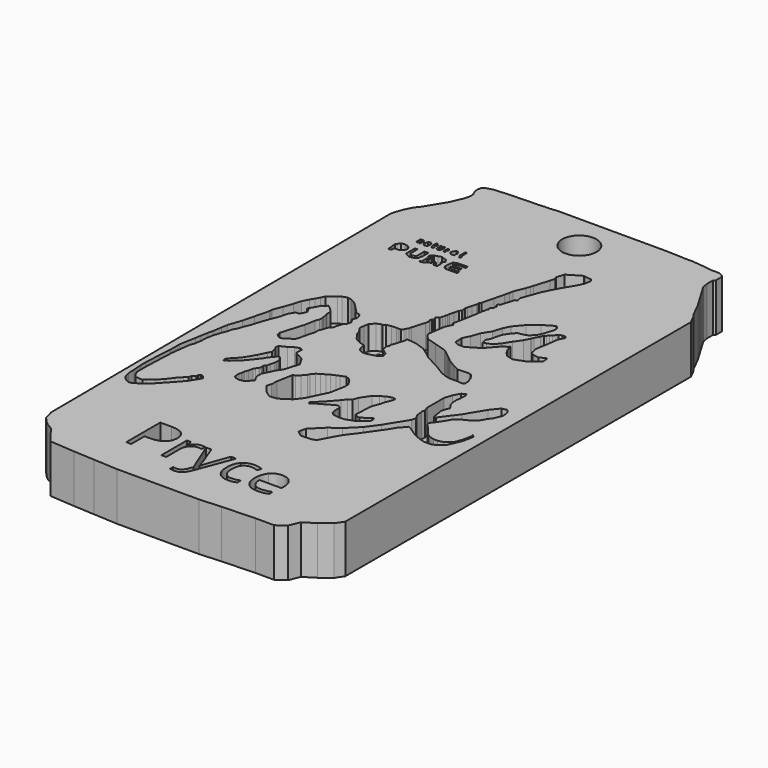
from build123d import *

# Parameters (mm, degrees)
F0_TEXT_SIZE = 6.2945538149
F1_DEPTH     = 2.54
F0_R         = 1.81247456
F2_DEPTH     = 5.08


# Not quite as in the source:
# - Text() gives the source's letters only with a copy of the font that has no kerning and outlines rounded to 1/6400 em; it was checked with that copy


with BuildPart() as f1:
    # F0 (on Top) → F1 (new body)
    with BuildSketch(Plane.XY):
        with Locations((-18.4478778392, -11.3192549907)):
            Text('Pryce', F0_TEXT_SIZE, font='Open Sans', text_align=(TextAlign.LEFT, TextAlign.BOTTOM))
        Polygon((-14.624286443, 6.6065290011), (-14.6113066003, 6.5750698559), (-14.9114299302, 4.9573605225), (-14.9448718876, 4.2598485015), (-15.1049830019, 3.7795153912), (-14.4143942744, 2.9255894478), (-13.7573806569, 2.4585989304), (-13.0635658279, 2.5119693018), (-12.5832324848, 2.7521359734), (-11.8360472843, 3.2724970952), (-11.2489731982, 4.0330248885), (-10.6618991122, 5.2605429664), (-10.2616213262, 6.0610985383), (-10.065051727, 7.1206378795), (-9.9613657221, 7.6809348539), (-9.9613657221, 8.0247446895), (-9.9935978651, 8.2181375474), (-10.3374077007, 8.7553402409), (-10.6274969876, 9.0131983161), (-10.9498184174, 9.142126888), (-11.4547898993, 8.9487340301), (-11.7878550664, 8.7983170524), (-12.1961291879, 8.626411669), (-12.5399390236, 8.4115304053), (-12.9267256707, 8.2181375474), (-13.2705355063, 7.9817688093), (-13.5713685304, 7.6164705679), (-13.6788096279, 7.42307771), (-14.0441069379, 6.9825709797), (-14.3879167736, 6.6924816929), align=None)
        Polygon((-13.0409123376, 6.1027472839), (-13.0857918411, 6.4729987644), (-13.0801750347, 6.4761852846), (-13.0689619109, 6.433729548), (-12.9118859768, 6.568366196), (-12.9343252629, 6.7030033097), (-12.9343252629, 6.7927609198), (-12.6426117495, 7.0171556436), (-12.205041945, 6.9947163574), (-11.9582079351, 6.9498373196), (-11.7450328544, 6.8376399577), (-11.5206381306, 6.568366196), (-11.3635621965, 6.489828229), (-11.3523425534, 6.2934826128), (-11.3579519093, 5.9400605969), (-11.3803921267, 5.8390833437), (-11.4028314129, 5.682006944), (-11.4925885573, 5.4744416848), (-11.5150287747, 5.4127331823), (-11.6496654227, 5.1434594207), (-12.0984548703, 4.6722302213), (-12.2555308044, 4.4702752493), (-12.3004103079, 4.3917368166), (-12.3901683837, 4.2234407738), (-12.5696836039, 3.9766067639), (-12.6987108961, 3.920508083), (-12.9511551932, 3.987826407), (-13.197989203, 4.2234412394), (-13.3101865649, 4.3973471038), (-13.2821369916, 4.6329614706), (-13.2540874183, 4.9639437348), (-13.0970114842, 5.2163880318), (-13.18676956, 5.2163880318), (-13.197989203, 5.3229755722), (-13.0745721981, 5.4407827556), align=None, mode=Mode.SUBTRACT)
        Polygon((-20.1555043459, 6.0734697618), (-20.7176841795, 5.5137774907), (-20.754635334, 5.265337415), (-20.6640698016, 5.0563374534), (-20.3923713416, 5.265337415), (-20.2739369124, 5.3280373104), (-20.0928039849, 5.5161374621), (-19.6121055633, 5.9132371098), (-19.4518715143, 6.0804365203), (-19.2777048796, 6.2964032404), (-18.9781393856, 6.6517028026), (-18.671605736, 7.0279026404), (-18.5253061354, 7.2438688949), (-18.3650720865, 7.4389353395), (-18.3650720865, 7.4946684763), (-18.0794391781, 7.8778350726), (-17.5848063082, 8.4909005091), (-17.4036733806, 8.4212338552), (-17.1110741794, 8.0032348633), (-17.1110741794, 7.8360345215), (-17.1110741794, 7.6131019741), (-17.1389412135, 7.3901684955), (-17.2583172873, 7.020606572), (-17.3409748822, 6.5750698559), (-17.5290741026, 6.3939369284), (-17.5012070686, 6.1222370714), (-17.5639074296, 5.8784037828), (-17.75200665, 5.6276042014), (-17.8704392165, 5.4325377569), (-17.9540403187, 4.9588046968), (-18.0028062314, 4.8473384231), (-18.0794391781, 4.6244054101), (-18.114272505, 4.457205534), (-18.1351732463, 4.2551723309), (-18.1909073144, 4.0252725594), (-18.2187724859, 3.7326728925), (-18.1769728661, 3.6421061959), (-18.1630402803, 3.4540065099), (-17.9819073528, 3.3007399179), (-17.7589729428, 3.2241067383), (-17.4454730004, 3.1962399371), (-17.1423219144, 3.2592936148), (-16.3936476487, 3.8831883856), (-16.4492409676, 3.9765057154), (-16.6443083435, 4.2760721408), (-16.7766753584, 4.6522719786), (-16.7740557998, 5.187679922), (-16.4422746748, 5.8366036974), (-16.2193421274, 6.3591031358), (-15.8156915272, 6.9102430428), (-15.5505435541, 7.7872681431), (-15.3276110068, 8.4560671821), (-15.8292111009, 9.3129668385), (-16.1636099219, 9.5358993858), (-16.5398102254, 9.7100660205), (-16.8602764606, 9.9120996892), (-16.8254431337, 10.6366323307), (-17.083209008, 10.7480986044), (-17.5778418779, 10.6017990038), (-18.0585421622, 10.2743655443), (-18.7552068383, 9.9329994991), (-18.8109409064, 9.5985997468), (-18.6642110338, 9.453726537), (-18.5322742909, 8.7695671245), (-18.7203735113, 8.4421345964), (-19.1244389862, 7.5991684571), (-19.7096392512, 6.6308025271), align=None)
        Polygon((-20.4632785171, 17.7643876523), (-20.2095806599, 17.9161417095), (-20.0275518, 18.1322433054), (-19.7358392179, 17.9161417095), (-19.3880274892, 17.5712574273), (-19.2085113376, 17.3917412758), (-19.2197300494, 16.9373415411), (-19.1243626177, 16.6400186718), (-19.0963130444, 16.3146462291), (-19.0417472463, 16.0316946908), (-19.0738718957, 15.7312210649), (-19.2253384739, 15.3273111209), (-19.4257468986, 14.2470799403), (-20.1641112822, 11.804805575), (-20.1018537056, 11.4819682355), (-19.9315026402, 11.3378688693), (-19.6667686105, 11.1288689077), (-19.3184353411, 11.2124690786), (-19.0397705883, 11.3587686792), (-18.8656039536, 11.5468688309), (-18.6496376991, 11.6165354848), (-18.3849036694, 11.895201169), (-18.196804449, 12.7312000841), (-18.0087033659, 13.4487664327), (-17.9181378335, 13.6508001015), (-17.9383958732, 14.1109345587), (-17.7718382329, 14.5355658606), (-17.5837371498, 15.0928990915), (-17.3062126196, 15.3241693663), (-17.231864767, 15.7249153367), (-17.0542709529, 16.2702649832), (-16.8104376644, 16.5419634432), (-16.7129039764, 16.9878304005), (-16.9183981761, 17.3327669933), (-17.0055031776, 17.3709969968), (-16.7895369232, 17.9161417095), (-16.9776361436, 18.4020623565), (-17.1796698123, 18.5553282499), (-17.4722690135, 18.5135286301), (-17.5976697356, 18.7573619187), (-18.653165549, 19.8301617056), (-19.2760806531, 20.1762262732), (-19.6913573891, 20.2454384416), (-20.2018022537, 20.0897101313), (-20.5046068877, 19.8993738741), (-21.2585731294, 19.2710691265), (-21.4562844485, 18.8265759498), (-21.6985289007, 18.4112992138), (-21.9321213663, 18.0219765753), (-22.2736951587, 17.3538995261), (-22.4944781512, 16.5771618485), (-22.8405427188, 15.6341381371), (-23.2212133706, 14.6392034367), (-23.2212133706, 14.3277458847), (-23.6091244797, 12.8109433288), (-23.914789253, 11.6157388134), (-24.3805292994, 10.2355387062), (-24.5034418927, 9.5730215691), (-24.6367733926, 8.6511746049), (-24.7707884197, 8.1271516241), (-24.9091346494, 7.3814448938), (-24.9975714833, 6.7610526457), (-25.3097963567, 5.0781141951), (-25.3097963567, 3.8123764098), (-25.4116076976, 2.5146363769), (-25.4894718528, 0.8456546348), (-25.4894718528, 0.1838220051), (-25.4116076976, -0.8108470356), (-25.3763237316, -1.6122754474), (-25.2426378429, -2.1516056731), (-24.9677542597, -2.5162470993), (-24.4183161264, -2.845908402), (-24.0084677935, -2.7518614661), (-23.6438252032, -2.5050272234), (-23.2904031873, -2.2357534617), (-22.6845387369, -1.7813541926), (-21.1651660502, -0.1317714487), (-20.6806752831, 0.4392341943), (-20.1382439994, 1.3322597274), (-20.0145021081, 1.5466390178), (-20.1875343919, 1.7975354567), (-20.3346125782, 1.8927031197), (-20.5422509462, 1.9100062782), (-20.6806752831, 1.7629291397), (-20.6806752831, 1.5293358592), (-20.7498893142, 1.4255166752), (-21.0094377398, 1.2438331032), (-21.0786499083, 0.9323754348), (-21.3728044182, 0.6987822126), (-21.8572933227, 0.1796862052), (-22.376390174, -0.5124418531), (-22.9560472071, -1.118053915), (-23.5097501427, -1.585240243), (-23.7450870523, -1.7813541926), (-24.5411440238, -1.7189012933), (-24.7647128999, -1.4563115546), (-24.9795932323, -0.9728290606), (-24.9795932323, -0.4893464502), (-24.9795932323, 0.316457852), (-24.8936414719, 2.5146363769), (-24.8506646603, 3.4429784864), (-24.6014371514, 5.4905763827), (-24.429531768, 5.9310826473), (-24.300603196, 6.7261429504), (-24.300603196, 7.2203697637), (-24.1470049222, 8.0482872776), (-23.8063763827, 9.1005796567), (-23.6749453002, 9.3576429668), (-23.623727262, 9.6055511385), (-23.5914960504, 9.841920808), (-23.3658701181, 10.1964743808), (-23.1187567115, 10.8948387206), (-22.9038763791, 11.3890646026), (-22.6204795463, 12.3101534486), (-22.3344415426, 13.1296021864), (-21.9321213663, 14.1395442188), (-21.7650067061, 14.8701397702), (-21.4038180918, 15.4721236742), (-20.9914352745, 15.5147835612), (-20.6906013191, 16.1594264209), (-20.948458463, 16.6751425713), (-21.0988745093, 16.6536532342), (-20.6866535317, 17.340691484), align=None)
        Polygon((-9.5739997969, 4.6030381121), (-10.4910627902, 3.6900329869), (-10.4620512575, 3.5761527251), (-10.4620512575, 3.5200540442), (-10.3666838259, 3.5312739201), (-10.2769257501, 3.5761527251), (-10.1254591718, 3.688350087), (-9.8730148748, 3.8454264868), (-9.6934996545, 3.95201426), (-9.3681272119, 4.1259201244), (-8.7678711861, 4.4737318531), (-8.6220148951, 4.5522698201), (-8.3863995969, 4.664467182), (-8.2517629489, 4.6869069338), (-8.0161485821, 4.5747095719), (-7.9488297924, 4.4288528152), (-7.9376101494, 4.1820188053), (-7.9488297924, 3.9912830107), (-7.8927315772, 3.677130444), (-7.859072648, 3.4527357202), (-7.6056825928, 3.2059017103), (-7.5108190067, 3.1607286073), (-7.307539694, 3.129107412), (-7.0455353707, 3.0974859837), (-6.7564267665, 3.079416696), (-6.2685562298, 3.129107412), (-5.9162052348, 3.2781788614), (-5.4804068059, 3.4207922872), (-5.2138781175, 3.6071261857), (-4.7017219476, 4.004185088), (-4.4716764241, 4.2033214122), (-4.4438098557, 4.4819880277), (-4.5204432681, 4.7745876946), (-4.7224764712, 4.7188540921), (-4.9941758625, 4.4401879422), (-5.1962090656, 4.356588237), (-5.5793751962, 4.119721707), (-5.8092749678, 4.1475882754), (-6.1436747201, 4.356588237), (-6.0740080662, 6.1191529967), (-5.9486082755, 6.5650194883), (-5.7256752625, 7.1502188221), (-5.6420755573, 7.4985516258), (-5.5236420594, 7.8190183267), (-5.4191425443, 8.0349845812), (-5.3285756148, 8.3763506263), (-5.3285756148, 8.5435509682), (-5.5306088179, 8.6271502078), (-5.8859083802, 8.5644507781), (-6.2830080278, 8.3763506263), (-6.673140917, 8.1673506647), (-7.1735936217, 7.7911512926), (-7.8087067232, 6.8297521211), (-8.0177066848, 6.3072526827), (-8.3590727299, 6.0216202401), (-8.6934724823, 5.6036203168), align=None)
        Polygon((-6.4959203971, 1.0680862335), (-7.7450601384, -0.1755262492), (-7.8824013472, -0.5878285156), (-7.8914361075, -0.9853526717), (-7.575223688, -1.2563917553), (-7.2770807892, -1.428049989), (-6.6536907107, -1.3964286773), (-6.0845082626, -1.3467381941), (-5.7482607663, -1.1509091128), (-5.6089274585, -0.8583095041), (-5.2675609477, -0.2173767425), (-4.8843948171, 0.479289185), (-4.4716764241, 1.1202218011), (-3.9090625942, 1.8447544426), (-2.4584615603, 3.9023284335), (-1.9673923962, 4.6953144483), (-1.5308865113, 5.1827458665), (-1.3781094458, 5.382811185), (-1.1453062762, 5.3136977367), (-0.5341977812, 4.8808292486), (0.0550852492, 4.5097991824), (0.808058132, 4.2006075382), (1.0808744701, 4.1387691163), (1.2409265619, 4.069655668), (1.4519045362, 4.069655668), (1.6919827322, 4.069655668), (2.0157247782, 4.0805684403), (2.3649295326, 4.2033214122), (2.5940951891, 4.3788473122), (3.0742518138, 4.7426023521), (3.387081204, 5.4191863164), (3.7071856204, 6.1576091684), (3.8672378287, 6.9069443271), (3.9108884521, 7.1797608398), (3.9145257324, 7.3361755349), (3.6562599707, 7.5544281863), (3.7362859584, 7.3085627519), (3.5494896583, 6.3745812513), (3.2559528481, 5.574026145), (2.9357306194, 5.3071742877), (2.5621380191, 5.0403224304), (2.0284343045, 4.9202390946), (1.6014714492, 4.9335816875), (1.1211381061, 5.080350209), (0.6941751344, 5.3472020663), (0.004460323, 6.2304427847), (-0.2592035162, 6.4828866161), (-0.4331094678, 6.7072813399), (-0.5092399145, 6.951796861), (-0.3096923756, 7.1504614316), (0.3747116425, 8.1602381542), (0.6495952257, 8.653906174), (1.1097851675, 9.0257488191), (2.0230300725, 9.4877434894), (2.4742805399, 9.8852738738), (2.8288345784, 10.4869408533), (3.1619002111, 10.9596792608), (3.5057100467, 11.8192043155), (3.3767814748, 12.5068239868), (3.0974359252, 12.8076579422), (2.5709769689, 12.7002168447), (1.8511251546, 11.8084605783), (0.6692788447, 9.8422979936), (-0.6457643467, 8.0773709342), (-0.8101447602, 8.0341128632), (-0.8534026565, 8.1119779497), (-0.88800909, 8.1811901182), (-1.0437379824, 9.2539889738), (-0.9053121903, 9.8336460069), (-0.7322800811, 10.0499354303), (-1.130253775, 10.620941408), (-1.2340729591, 10.9670050442), (-1.2686793925, 11.6331782192), (-1.1994665256, 11.9532877579), (-1.156208571, 12.6454159617), (-1.3032857096, 12.9136154428), (-1.683956245, 12.680022046), (-2.047323389, 12.0225008577), (-2.306871349, 11.2179024145), (-2.306871349, 10.5776842684), (-2.306871349, 9.3837631866), (-2.306871349, 9.0030925348), (-2.151142573, 8.5359057412), (-2.211703686, 8.1552360207), (-2.1259179339, 7.4634985067), (-1.8573165871, 6.969272159), (-1.9540130161, 6.4965337515), (-3.3292525914, 4.2725135572), (-4.2559751181, 3.0073651436), (-5.4673198611, 1.801380422), align=None)
        Polygon((-8.3126790669, 34.6074029803), (-8.5634384304, 33.7779708207), (-8.4576277141, 33.6387456779), (-8.4563963125, 33.4593554644), (-8.565570089, 33.0324662643), (-9.0527144692, 31.4491625604), (-9.1438563541, 31.1476942152), (-9.2830456478, 30.7437833399), (-9.7441114485, 29.5993704349), (-9.8226498812, 29.2235091329), (-9.9271811918, 28.7110497152), (-10.1888252151, 27.6879742894), (-10.4962536496, 26.4858735394), (-10.4910627902, 26.3679700631), (-10.6509367006, 26.2347419007), (-10.5799818411, 26.1156391352), (-10.6384458912, 25.9256208353), (-10.769763142, 25.491265167), (-10.8820305236, 25.0522794112), (-10.9558422118, 24.7636623681), (-10.913762163, 24.6164460853), (-10.8997439966, 24.2980420589), (-11.0629596188, 24.1172267462), (-11.185686636, 23.6373419248), (-11.3036539406, 23.1760684401), (-11.3260932267, 22.9348447174), (-11.3925919681, 22.738418241), (-11.4660311696, 22.4512576879), (-11.5504879504, 22.171901539), (-11.8395954764, 21.9443800978), (-11.7300031707, 21.8128692359), (-11.7138029971, 21.6744998852), (-11.8395954764, 21.5696728948), (-11.9151296094, 21.2743207812), (-11.8019562101, 21.2453775159), (-11.7804920301, 21.1340747774), (-11.869258746, 20.7286904829), (-12.2741600499, 19.3894058466), (-12.3414788395, 19.120130688), (-12.4633380084, 18.867270008), (-12.5434342772, 18.7106113881), (-12.7117298543, 18.5367055237), (-12.8968553618, 18.5367055237), (-13.2166184485, 18.5479242355), (-13.6747442755, 18.5213295529), (-14.2171129882, 18.4167364419), (-14.4143942744, 18.2523354888), (-14.6107394248, 18.2523354888), (-14.9866007268, 18.0728193372), (-15.3995410008, 17.6408607513), (-15.4858790338, 17.1471927315), (-15.5435165947, 16.6064269245), (-15.3995410008, 16.433656087), (-15.129315725, 15.9800637904), (-15.0763588026, 15.7054550946), (-14.509761706, 14.9312941357), (-14.2460977659, 14.7517779842), (-13.8027653814, 14.5654321793), (-13.3429095149, 14.4264055416), (-13.2346283644, 13.8649124606), (-13.0573342346, 13.5673116855), (-12.6528963447, 13.3605310693), (-12.2545957565, 13.3605310693), (-11.4214839913, 13.5743296974), (-10.8857871965, 13.8934683055), (-10.9983412549, 14.3703082576), (-11.6767790169, 14.8639772087), (-11.7440968752, 15.4586229473), (-11.6094602272, 15.6830176711), (-11.6930775197, 15.8593941689), (-11.5213871949, 16.1951996906), (-11.2422769889, 17.1184074134), (-11.1880693585, 17.4617245793), (-10.9983412549, 17.4617245793), (-10.212328285, 17.3758957535), (-9.1281700879, 17.0099921525), (-8.5860919207, 16.6169852018), (-7.7543499912, 15.9858464067), (-6.4606027193, 15.3243805433), (-5.7285217531, 14.8797083547), (-5.2387579344, 14.5796732977), (-4.7328183427, 14.3673596904), (-4.172670655, 14.2228053883), (-3.1698255334, 14.2228053883), (-2.791371457, 14.1743155537), (-2.5757015937, 14.35404031), (-2.5780566502, 14.6971242502), (-2.7144698237, 15.1888835414), (-2.9808814856, 15.6360744166), (-3.1489883779, 15.8378028329), (-3.4577118056, 15.9311381218), (-4.623724381, 15.8798028466), (-5.2595826652, 16.2049038598), (-6.0471831821, 16.6832990944), (-6.756614428, 17.2716081142), (-7.6047767337, 17.9161417095), (-8.8898812928, 18.3046629376), (-9.8798424006, 18.6039544642), (-10.2280915304, 18.9104281538), (-10.4681514204, 19.3133857101), (-10.2055160521, 21.1895945882), (-9.8464093118, 21.8919639639), (-10.065051727, 22.0037512481), (-9.5801549032, 24.5290119201), (-9.5024109221, 25.2584492622), (-9.4114554086, 25.4363472518), (-9.421107778, 25.6555879974), (-9.2830456478, 25.9256208353), (-9.3802224422, 26.0887389788), (-9.2786931039, 26.1733466996), (-9.1650243849, 26.2680705637), (-9.090193182, 26.7056394368), (-9.2603927478, 26.8514975905), (-9.2643508225, 27.0925729386), (-9.090193182, 27.03992046), (-8.6557937713, 28.4767754443), (-8.438963443, 28.6059509963), (-8.542782627, 28.9952736348), (-7.843706755, 30.9560261331), (-7.085440597, 32.4391030801), (-6.4096620912, 33.5516632854), (-6.1940371231, 33.9733996588), (-6.0096010566, 34.3341343105), (-5.8784423407, 35.0494985358), (-6.037467625, 35.3164337575), (-6.1698341742, 35.3164337575), (-6.7144366423, 35.3842654844), (-6.9096128755, 35.4432724416), align=None)
        Polygon((-14.024060809, 16.0090131449), (-14.2227048054, 16.2473861128), (-14.3074673342, 16.4911487616), (-14.3786463886, 16.860248521), (-14.4616509004, 17.239703682), (-14.4804976881, 17.6677834243), (-14.2549695447, 17.7623592317), (-13.7748131528, 17.8169235587), (-13.294656761, 17.8605746478), (-13.0372691302, 17.9550269006), (-12.7746119231, 17.8878542497), (-12.7556817606, 17.7896916866), (-12.8482754727, 17.3078885362), (-13.0062680691, 16.6901089251), (-13.2987415418, 16.3032896817), (-13.5770635679, 16.0957276821), (-13.7421693653, 16.0155333579), (-13.9261345659, 15.9589455093), align=None, mode=Mode.SUBTRACT)
        Polygon((-2.9255773406, 26.918547228), (-3.0908517074, 27.03992046), (-4.2187681199, 26.3679700631), (-5.1508066244, 25.5947168916), (-5.9595149942, 24.6384963393), (-6.3162512995, 23.9407632478), (-6.6027877955, 22.9929917214), (-7.1628494188, 22.1028998494), (-7.4744271114, 21.189654246), (-7.843706755, 20.4673879012), (-7.804661861, 19.5805350076), (-7.4959155172, 19.4061398506), (-7.1735936217, 19.3524211645), (-6.6901110113, 19.3631649017), (-5.3732738056, 20.1476638887), (-4.9710618332, 20.6309631467), (-4.3801385909, 21.2970953435), (-3.8214477245, 21.6838810593), (-3.7485628504, 21.8038742372), (-3.6065666936, 21.5979292989), (-3.6065666936, 21.2111417204), (-3.3010091144, 20.6982416459), (-2.8974588495, 20.2978979796), (-2.2098391782, 20.1367363334), (-1.0007828241, 20.5557551235), (-0.3774818159, 21.0751722551), (0, 21.3897402078), (-0.0261788142, 21.9843571922), (-0.2006201078, 22.0289692713), (-0.7254455944, 21.7163071892), (-1.4577549882, 21.8450408429), (-1.7156124813, 22.0706667751), (-1.77424332, 22.3746976255), (-1.8445411697, 22.6723346859), (-1.8015649403, 23.1450721622), (-1.668242272, 23.8637011498), (-1.550792018, 24.6994066983), (-1.4875495108, 25.214381516), (-1.2481315061, 25.6390087306), (-1.1803717352, 25.83325468), (-1.3565472327, 26.0184649378), (-1.6501729842, 26.0320156813), (-1.9709027838, 25.8919801563), (-2.0838356577, 25.7293563336), (-2.3187363986, 25.5215596408), (-2.4994290434, 25.3499019891), (-2.6394659653, 25.1466222107), (-2.797572175, 25.0427238643), (-2.9150224291, 24.7355457395), (-3.222200321, 24.2115370929), (-3.3125467598, 23.9856708795), (-3.3486853354, 23.9043589681), (-3.6329326326, 23.3484056141), (-4.1800593026, 22.5667897612), (-4.6500945727, 21.7929525761), (-4.9414001405, 21.4766878635), (-5.1508066244, 21.2344434112), (-5.6335283443, 21.0095010698), (-6.0141985305, 20.9575910121), (-6.0661081225, 21.1652312428), (-6.1093661934, 21.4766878635), (-5.9103793465, 21.7881463468), (-5.606696517, 22.9756011037), (-5.3134192713, 23.4492532909), (-4.8375814222, 24.0289121866), (-4.3184850365, 24.1154283285), (-3.7993891165, 24.2980420589), (-3.2716414426, 24.8940717429), (-3.0380480457, 25.4650767893), (-2.7941309582, 26.2578496174), (-2.7698485646, 26.6070887446), (-2.7871516068, 26.7455149442), align=None)
    extrude(amount=F1_DEPTH)


with BuildPart() as f2:
    # F0 (on Top) → F2 (new body)
    with BuildSketch(Plane.XY):
        Polygon((-26.1796228588, 34.6074029803), (-26.3012740761, 34.205019474), (-25.9908363223, -11.0194599256), (-25.7235337049, -12.0254354551), (-25.2498015761, -12.554901652), (-24.7691012919, -12.952000834), (-24.2466013879, -13.2237011567), (-22.8281021118, -15.0916650891), (-20.1595854014, -15.2918035164), (-17.9580561817, -15.4118873179), (-15.4246796457, -15.5500719408), (-12.9279000685, -15.5500719408), (-10.8464555815, -15.5500719408), (-9.0185198933, -15.5500719408), (-6.736936979, -15.5500719408), (-4.5220665634, -15.4118873179), (-1.0007828241, -15.2739165351), (0.9544302593, -15.2739165351), (1.8823278369, -14.611132443), (2.3462767713, -13.4843997657), (3.5061491653, -12.7553371713), (4.5997425914, -11.9102876633), (5.1299701445, -11.1149465665), (5.1299701445, -10.3030363098), (5.1299701445, -6.0831848532), (5.1299701445, -5.6025036611), (5.1299701445, 0.4914481542), (5.1299701445, 34.4898588955), (4.697042983, 35.3593826294), (4.482162185, 35.6172397733), (3.6763579119, 37.2288487852), (3.0746906996, 38.2387898862), (2.0099615683, 40.0260132701), (1.8928443315, 40.6884364784), (1.8928443315, 41.1182008684), (1.8928443315, 41.4620116353), (2.0682715006, 41.6082008373), (2.0682715006, 41.9347472489), (2.0682715006, 42.4152649939), (1.9506843017, 42.5563697345), (1.489731716, 42.7963659167), (0.6548750098, 42.7963659167), (-0.4625069851, 42.9459773004), (-1.543660881, 43.0526062846), (-2.396360971, 43.0526062846), (-4.1298102587, 43.1367568672), (-5.1508066244, 43.1367568672), (-6.5364441834, 43.1367568672), (-8.6120953783, 43.1367568672), (-9.4030871987, 43.1367568672), (-10.065051727, 43.1367568672), (-11.0804382712, 43.1367568672), (-13.2346283644, 43.1367568672), (-14.730071649, 43.1367568672), (-15.7961584628, 43.1367568672), (-16.564104706, 43.0526062846), (-17.1423219144, 43.0526062846), (-17.7792627364, 42.9885946214), (-18.7730714679, 42.9885946214), (-20.2095806599, 42.925350368), (-21.2255993903, 42.880618774), (-22.319169715, 42.7963659167), (-23.0600088835, 42.6046214998), (-23.3068708686, 42.4575547429), (-23.3915168792, 42.0124307275), (-23.3761685055, 41.6638128109), (-23.2007820159, 41.210219264), (-23.1241000749, 41.1182008684), (-23.1241000749, 40.5706912279), (-23.3017597347, 39.9704352021), (-23.5429834574, 39.4150614738), (-23.8010380417, 38.82041201), (-24.261046201, 38.063082844), (-24.6425177902, 37.4403856695), (-25.0899949594, 36.7099439359), (-25.5008284003, 36.1893847585), (-25.8822999895, 35.4432724416), (-26.0449871421, 35.02253443), align=None)
        with BuildLine():
            add(Edge.make_bspline(
                [(-16.6647487663, -6.8255336813), (-14.9809556209, -6.8255336813), (-14.9809556209, -8.13460417)],
                knots=[0, 0, 0, 1, 1, 1], degree=2))
            add(Edge.make_bspline(
                [(-14.9809556209, -8.13460417), (-14.9809556209, -8.8171698493), (-15.4466542508, -9.1845160758)],
                knots=[0, 0, 0, 1, 1, 1], degree=2))
            add(Edge.make_bspline(
                [(-15.4466542508, -9.1845160758), (-15.9123528807, -9.5518623023), (-16.7788375542, -9.5518623023)],
                knots=[0, 0, 0, 1, 1, 1], degree=2))
            Line((-16.7788375542, -9.5518623023), (-17.3079734843, -9.5518623023))
            Line((-17.3079734843, -9.5518623023), (-17.3079734843, -11.3192549907))
            Line((-17.3079734843, -11.3192549907), (-17.8302247461, -11.3192549907))
            Line((-17.8302247461, -11.3192549907), (-17.8302247461, -6.8255336813))
            Line((-17.8302247461, -6.8255336813), (-16.6647487663, -6.8255336813))
        make_face(mode=Mode.SUBTRACT)
        with BuildLine():
            add(Edge.make_bspline(
                [(-13.1614361588, -8.0672327737), (-12.8968681937, -7.8887231616), (-12.5801734549, -7.8887231616)],
                knots=[0, 0, 0, 1, 1, 1], degree=2))
            add(Edge.make_bspline(
                [(-12.5801734549, -7.8887231616), (-12.3559299753, -7.8887231616), (-12.1779121252, -7.9260970748)],
                knots=[0, 0, 0, 1, 1, 1], degree=2))
            Line((-12.1779121252, -7.9260970748), (-12.2487258556, -8.399172135))
            add(Edge.make_bspline(
                [(-12.2487258556, -8.399172135), (-12.4572329507, -8.3529465054), (-12.6175473682, -8.3529465054)],
                knots=[0, 0, 0, 1, 1, 1], degree=2))
            add(Edge.make_bspline(
                [(-12.6175473682, -8.3529465054), (-13.0266933662, -8.3529465054), (-13.3168329561, -8.6848858667)],
                knots=[0, 0, 0, 1, 1, 1], degree=2))
            add(Edge.make_bspline(
                [(-13.3168329561, -8.6848858667), (-13.606972546, -9.0168252281), (-13.606972546, -9.511537817)],
                knots=[0, 0, 0, 1, 1, 1], degree=2))
            Line((-13.606972546, -9.511537817), (-13.606972546, -11.3192549907))
            Line((-13.606972546, -11.3192549907), (-14.1174215194, -11.3192549907))
            Line((-14.1174215194, -11.3192549907), (-14.1174215194, -7.9506851757))
            Line((-14.1174215194, -7.9506851757), (-13.696473233, -7.9506851757))
            Line((-13.696473233, -7.9506851757), (-13.637461791, -8.574239413))
            Line((-13.637461791, -8.574239413), (-13.6128736902, -8.574239413))
            add(Edge.make_bspline(
                [(-13.6128736902, -8.574239413), (-13.4260041238, -8.2457423858), (-13.1614361588, -8.0672327737)],
                knots=[0, 0, 0, 1, 1, 1], degree=2))
        make_face(mode=Mode.SUBTRACT)
        Polygon((-20.0275518, 18.1322433054), (-20.2095806599, 17.9161417095), (-20.4632785171, 17.7643876523), (-20.6866535317, 17.340691484), (-21.0988745093, 16.6536532342), (-20.948458463, 16.6751425713), (-20.6906013191, 16.1594264209), (-20.9914352745, 15.5147835612), (-21.4038180918, 15.4721236742), (-21.7650067061, 14.8701397702), (-21.9321213663, 14.1395442188), (-22.3344415426, 13.1296021864), (-22.6204795463, 12.3101534486), (-22.9038763791, 11.3890646026), (-23.1187567115, 10.8948387206), (-23.3658701181, 10.1964743808), (-23.5914960504, 9.841920808), (-23.623727262, 9.6055511385), (-23.6749453002, 9.3576429668), (-23.8063763827, 9.1005796567), (-24.1470049222, 8.0482872776), (-24.300603196, 7.2203697637), (-24.300603196, 6.7261429504), (-24.429531768, 5.9310826473), (-24.6014371514, 5.4905763827), (-24.8506646603, 3.4429784864), (-24.8936414719, 2.5146363769), (-24.9795932323, 0.316457852), (-24.9795932323, -0.4893464502), (-24.9795932323, -0.9728290606), (-24.7647128999, -1.4563115546), (-24.5411440238, -1.7189012933), (-23.7450870523, -1.7813541926), (-23.5097501427, -1.585240243), (-22.9560472071, -1.118053915), (-22.376390174, -0.5124418531), (-21.8572933227, 0.1796862052), (-21.3728044182, 0.6987822126), (-21.0786499083, 0.9323754348), (-21.0094377398, 1.2438331032), (-20.7498893142, 1.4255166752), (-20.6806752831, 1.5293358592), (-20.6806752831, 1.7629291397), (-20.5422509462, 1.9100062782), (-20.3346125782, 1.8927031197), (-20.1875343919, 1.7975354567), (-20.0145021081, 1.5466390178), (-20.1382439994, 1.3322597274), (-20.6806752831, 0.4392341943), (-21.1651660502, -0.1317714487), (-22.6845387369, -1.7813541926), (-23.2904031873, -2.2357534617), (-23.6438252032, -2.5050272234), (-24.0084677935, -2.7518614661), (-24.4183161264, -2.845908402), (-24.9677542597, -2.5162470993), (-25.2426378429, -2.1516056731), (-25.3763237316, -1.6122754474), (-25.4116076976, -0.8108470356), (-25.4894718528, 0.1838220051), (-25.4894718528, 0.8456546348), (-25.4116076976, 2.5146363769), (-25.3097963567, 3.8123764098), (-25.3097963567, 5.0781141951), (-24.9975714833, 6.7610526457), (-24.9091346494, 7.3814448938), (-24.7707884197, 8.1271516241), (-24.6367733926, 8.6511746049), (-24.5034418927, 9.5730215691), (-24.3805292994, 10.2355387062), (-23.914789253, 11.6157388134), (-23.6091244797, 12.8109433288), (-23.2212133706, 14.3277458847), (-23.2212133706, 14.6392034367), (-22.8405427188, 15.6341381371), (-22.4944781512, 16.5771618485), (-22.2736951587, 17.3538995261), (-21.9321213663, 18.0219765753), (-21.6985289007, 18.4112992138), (-21.4562844485, 18.8265759498), (-21.2585731294, 19.2710691265), (-20.5046068877, 19.8993738741), (-20.2018022537, 20.0897101313), (-19.6913573891, 20.2454384416), (-19.2760806531, 20.1762262732), (-18.653165549, 19.8301617056), (-17.5976697356, 18.7573619187), (-17.4722690135, 18.5135286301), (-17.1796698123, 18.5553282499), (-16.9776361436, 18.4020623565), (-16.7895369232, 17.9161417095), (-17.0055031776, 17.3709969968), (-16.9183981761, 17.3327669933), (-16.7129039764, 16.9878304005), (-16.8104376644, 16.5419634432), (-17.0542709529, 16.2702649832), (-17.231864767, 15.7249153367), (-17.3062126196, 15.3241693663), (-17.5837371498, 15.0928990915), (-17.7718382329, 14.5355658606), (-17.9383958732, 14.1109345587), (-17.9181378335, 13.6508001015), (-18.0087033659, 13.4487664327), (-18.196804449, 12.7312000841), (-18.3849036694, 11.895201169), (-18.6496376991, 11.6165354848), (-18.8656039536, 11.5468688309), (-19.0397705883, 11.3587686792), (-19.3184353411, 11.2124690786), (-19.6667686105, 11.1288689077), (-19.9315026402, 11.3378688693), (-20.1018537056, 11.4819682355), (-20.1641112822, 11.804805575), (-19.4257468986, 14.2470799403), (-19.2253384739, 15.3273111209), (-19.0738718957, 15.7312210649), (-19.0417472463, 16.0316946908), (-19.0963130444, 16.3146462291), (-19.1243626177, 16.6400186718), (-19.2197300494, 16.9373415411), (-19.2085113376, 17.3917412758), (-19.3880274892, 17.5712574273), (-19.7358392179, 17.9161417095), align=None, mode=Mode.SUBTRACT)
        Polygon((-14.9114299302, 4.9573605225), (-14.6113066003, 6.5750698559), (-14.624286443, 6.6065290011), (-14.3879167736, 6.6924816929), (-14.0441069379, 6.9825709797), (-13.6788096279, 7.42307771), (-13.5713685304, 7.6164705679), (-13.2705355063, 7.9817688093), (-12.9267256707, 8.2181375474), (-12.5399390236, 8.4115304053), (-12.1961291879, 8.626411669), (-11.7878550664, 8.7983170524), (-11.4547898993, 8.9487340301), (-10.9498184174, 9.142126888), (-10.6274969876, 9.0131983161), (-10.3374077007, 8.7553402409), (-9.9935978651, 8.2181375474), (-9.9613657221, 8.0247446895), (-9.9613657221, 7.6809348539), (-10.065051727, 7.1206378795), (-10.2616213262, 6.0610985383), (-10.6618991122, 5.2605429664), (-11.2489731982, 4.0330248885), (-11.8360472843, 3.2724970952), (-12.5832324848, 2.7521359734), (-13.0635658279, 2.5119693018), (-13.7573806569, 2.4585989304), (-14.4143942744, 2.9255894478), (-15.1049830019, 3.7795153912), (-14.9448718876, 4.2598485015), align=None, mode=Mode.SUBTRACT)
        Polygon((-20.754635334, 5.265337415), (-20.7176841795, 5.5137774907), (-20.1555043459, 6.0734697618), (-19.7096392512, 6.6308025271), (-19.1244389862, 7.5991684571), (-18.7203735113, 8.4421345964), (-18.5322742909, 8.7695671245), (-18.6642110338, 9.453726537), (-18.8109409064, 9.5985997468), (-18.7552068383, 9.9329994991), (-18.0585421622, 10.2743655443), (-17.5778418779, 10.6017990038), (-17.083209008, 10.7480986044), (-16.8254431337, 10.6366323307), (-16.8602764606, 9.9120996892), (-16.5398102254, 9.7100660205), (-16.1636099219, 9.5358993858), (-15.8292111009, 9.3129668385), (-15.3276110068, 8.4560671821), (-15.5505435541, 7.7872681431), (-15.8156915272, 6.9102430428), (-16.2193421274, 6.3591031358), (-16.4422746748, 5.8366036974), (-16.7740557998, 5.187679922), (-16.7766753584, 4.6522719786), (-16.6443083435, 4.2760721408), (-16.4492409676, 3.9765057154), (-16.3936476487, 3.8831883856), (-17.1423219144, 3.2592936148), (-17.4454730004, 3.1962399371), (-17.7589729428, 3.2241067383), (-17.9819073528, 3.3007399179), (-18.1630402803, 3.4540065099), (-18.1769728661, 3.6421061959), (-18.2187724859, 3.7326728925), (-18.1909073144, 4.0252725594), (-18.1351732463, 4.2551723309), (-18.114272505, 4.457205534), (-18.0794391781, 4.6244054101), (-18.0028062314, 4.8473384231), (-17.9540403187, 4.9588046968), (-17.8704392165, 5.4325377569), (-17.75200665, 5.6276042014), (-17.5639074296, 5.8784037828), (-17.5012070686, 6.1222370714), (-17.5290741026, 6.3939369284), (-17.3409748822, 6.5750698559), (-17.2583172873, 7.020606572), (-17.1389412135, 7.3901684955), (-17.1110741794, 7.6131019741), (-17.1110741794, 7.8360345215), (-17.1110741794, 8.0032348633), (-17.4036733806, 8.4212338552), (-17.5848063082, 8.4909005091), (-18.0794391781, 7.8778350726), (-18.3650720865, 7.4946684763), (-18.3650720865, 7.4389353395), (-18.5253061354, 7.2438688949), (-18.671605736, 7.0279026404), (-18.9781393856, 6.6517028026), (-19.2777048796, 6.2964032404), (-19.4518715143, 6.0804365203), (-19.6121055633, 5.9132371098), (-20.0928039849, 5.5161374621), (-20.2739369124, 5.3280373104), (-20.3923713416, 5.265337415), (-20.6640698016, 5.0563374534), align=None, mode=Mode.SUBTRACT)
        with BuildLine():
            Line((-10.7232800795, -11.3379419473), (-12.0825102939, -7.9506851757))
            Line((-12.0825102939, -7.9506851757), (-11.5346874072, -7.9506851757))
            Line((-11.5346874072, -7.9506851757), (-10.797044382, -9.8715076132))
            add(Edge.make_bspline(
                [(-10.797044382, -9.8715076132), (-10.5550974698, -10.5294851917), (-10.4960860278, -10.8215918297)],
                knots=[0, 0, 0, 1, 1, 1], degree=2))
            Line((-10.4960860278, -10.8215918297), (-10.4714979269, -10.8215918297))
            add(Edge.make_bspline(
                [(-10.4714979269, -10.8215918297), (-10.4321569656, -10.6642279843), (-10.3042988412, -10.2845877073)],
                knots=[0, 0, 0, 1, 1, 1], degree=2))
            add(Edge.make_bspline(
                [(-10.3042988412, -10.2845877073), (-10.1764407169, -9.9049474304), (-9.4692869367, -7.9506851757)],
                knots=[0, 0, 0, 1, 1, 1], degree=2))
            Line((-9.4692869367, -7.9506851757), (-8.922447574, -7.9506851757))
            Line((-8.922447574, -7.9506851757), (-10.3701949515, -11.7864289066))
            add(Edge.make_bspline(
                [(-10.3701949515, -11.7864289066), (-10.5855867148, -12.354905798), (-10.8727757326, -12.5934103762)],
                knots=[0, 0, 0, 1, 1, 1], degree=2))
            add(Edge.make_bspline(
                [(-10.8727757326, -12.5934103762), (-11.1599647504, -12.8319149543), (-11.5779624647, -12.8319149543)],
                knots=[0, 0, 0, 1, 1, 1], degree=2))
            add(Edge.make_bspline(
                [(-11.5779624647, -12.8319149543), (-11.8120411847, -12.8319149543), (-12.0392352364, -12.7788046565)],
                knots=[0, 0, 0, 1, 1, 1], degree=2))
            Line((-12.0392352364, -12.7788046565), (-12.0392352364, -12.3706421826))
            add(Edge.make_bspline(
                [(-12.0392352364, -12.3706421826), (-11.8700691027, -12.4070325718), (-11.6615620076, -12.4070325718)],
                knots=[0, 0, 0, 1, 1, 1], degree=2))
            add(Edge.make_bspline(
                [(-11.6615620076, -12.4070325718), (-11.1353766496, -12.4070325718), (-10.9111331699, -11.8169181517)],
                knots=[0, 0, 0, 1, 1, 1], degree=2))
            Line((-10.9111331699, -11.8169181517), (-10.7232800795, -11.3379419473))
        make_face(mode=Mode.SUBTRACT)
        with BuildLine():
            add(Edge.make_bspline(
                [(-6.1784155204, -11.2051662028), (-6.5157642639, -11.3812170048), (-7.0291638094, -11.3812170048)],
                knots=[0, 0, 0, 1, 1, 1], degree=2))
            add(Edge.make_bspline(
                [(-7.0291638094, -11.3812170048), (-7.7609056904, -11.3812170048), (-8.1621834961, -10.9307629974)],
                knots=[0, 0, 0, 1, 1, 1], degree=2))
            add(Edge.make_bspline(
                [(-8.1621834961, -10.9307629974), (-8.5634613018, -10.48030899), (-8.5634613018, -9.6561158499)],
                knots=[0, 0, 0, 1, 1, 1], degree=2))
            add(Edge.make_bspline(
                [(-8.5634613018, -9.6561158499), (-8.5634613018, -8.8112687051), (-8.1557905899, -8.3499959333)],
                knots=[0, 0, 0, 1, 1, 1], degree=2))
            add(Edge.make_bspline(
                [(-8.1557905899, -8.3499959333), (-7.748119878, -7.8887231616), (-6.9957239923, -7.8887231616)],
                knots=[0, 0, 0, 1, 1, 1], degree=2))
            add(Edge.make_bspline(
                [(-6.9957239923, -7.8887231616), (-6.752793556, -7.8887231616), (-6.5098631197, -7.9413416974)],
                knots=[0, 0, 0, 1, 1, 1], degree=2))
            add(Edge.make_bspline(
                [(-6.5098631197, -7.9413416974), (-6.2669326834, -7.9939602332), (-6.1292393187, -8.0647739636)],
                knots=[0, 0, 0, 1, 1, 1], degree=2))
            Line((-6.1292393187, -8.0647739636), (-6.28561964, -8.4975245383))
            add(Edge.make_bspline(
                [(-6.28561964, -8.4975245383), (-6.4547857738, -8.42966138), (-6.6544411526, -8.3854027985)],
                knots=[0, 0, 0, 1, 1, 1], degree=2))
            add(Edge.make_bspline(
                [(-6.6544411526, -8.3854027985), (-6.8540965314, -8.341144217), (-7.0075262807, -8.341144217)],
                knots=[0, 0, 0, 1, 1, 1], degree=2))
            add(Edge.make_bspline(
                [(-7.0075262807, -8.341144217), (-8.0343253717, -8.341144217), (-8.0343253717, -9.6502147057)],
                knots=[0, 0, 0, 1, 1, 1], degree=2))
            add(Edge.make_bspline(
                [(-8.0343253717, -9.6502147057), (-8.0343253717, -10.2708183709), (-7.7840185052, -10.6027577322)],
                knots=[0, 0, 0, 1, 1, 1], degree=2))
            add(Edge.make_bspline(
                [(-7.7840185052, -10.6027577322), (-7.5337116386, -10.9346970935), (-7.0419496219, -10.9346970935)],
                knots=[0, 0, 0, 1, 1, 1], degree=2))
            add(Edge.make_bspline(
                [(-7.0419496219, -10.9346970935), (-6.6210013355, -10.9346970935), (-6.1784155204, -10.7537286714)],
                knots=[0, 0, 0, 1, 1, 1], degree=2))
            Line((-6.1784155204, -10.7537286714), (-6.1784155204, -11.2051662028))
        make_face(mode=Mode.SUBTRACT)
        with BuildLine():
            add(Edge.make_bspline(
                [(-3.3734049766, -11.330073755), (-3.6143683649, -11.3812170048), (-3.9556512045, -11.3812170048)],
                knots=[0, 0, 0, 1, 1, 1], degree=2))
            add(Edge.make_bspline(
                [(-3.9556512045, -11.3812170048), (-4.702145946, -11.3812170048), (-5.1344047587, -10.9258453772)],
                knots=[0, 0, 0, 1, 1, 1], degree=2))
            add(Edge.make_bspline(
                [(-5.1344047587, -10.9258453772), (-5.5666635715, -10.4704737497), (-5.5666635715, -9.6630005181)],
                knots=[0, 0, 0, 1, 1, 1], degree=2))
            add(Edge.make_bspline(
                [(-5.5666635715, -9.6630005181), (-5.5666635715, -8.8476590943), (-5.1653857658, -8.3681911279)],
                knots=[0, 0, 0, 1, 1, 1], degree=2))
            add(Edge.make_bspline(
                [(-5.1653857658, -8.3681911279), (-4.7641079601, -7.8887231616), (-4.087443425, -7.8887231616)],
                knots=[0, 0, 0, 1, 1, 1], degree=2))
            add(Edge.make_bspline(
                [(-4.087443425, -7.8887231616), (-3.4550374714, -7.8887231616), (-3.0862159588, -8.3052455898)],
                knots=[0, 0, 0, 1, 1, 1], degree=2))
            add(Edge.make_bspline(
                [(-3.0862159588, -8.3052455898), (-2.7173944462, -8.721768018), (-2.7173944462, -9.4043336973)],
                knots=[0, 0, 0, 1, 1, 1], degree=2))
            Line((-2.7173944462, -9.4043336973), (-2.7173944462, -9.7269295803))
            Line((-2.7173944462, -9.7269295803), (-5.0375276414, -9.7269295803))
            add(Edge.make_bspline(
                [(-5.0375276414, -9.7269295803), (-5.0217912569, -10.3199945726), (-4.7375528112, -10.627345833)],
                knots=[0, 0, 0, 1, 1, 1], degree=2))
            add(Edge.make_bspline(
                [(-4.7375528112, -10.627345833), (-4.4533143655, -10.9346970935), (-3.9369642479, -10.9346970935)],
                knots=[0, 0, 0, 1, 1, 1], degree=2))
            add(Edge.make_bspline(
                [(-3.9369642479, -10.9346970935), (-3.3930754573, -10.9346970935), (-2.8619724792, -10.7075030418)],
                knots=[0, 0, 0, 1, 1, 1], degree=2))
            Line((-2.8619724792, -10.7075030418), (-2.8619724792, -11.1628746693))
            add(Edge.make_bspline(
                [(-2.8619724792, -11.1628746693), (-3.1324415884, -11.2789305053), (-3.3734049766, -11.330073755)],
                knots=[0, 0, 0, 1, 1, 1], degree=2))
        make_face(mode=Mode.SUBTRACT)
        Polygon((-10.4620512575, 3.5761527251), (-10.4910627902, 3.6900329869), (-9.5739997969, 4.6030381121), (-8.6934724823, 5.6036203168), (-8.3590727299, 6.0216202401), (-8.0177066848, 6.3072526827), (-7.8087067232, 6.8297521211), (-7.1735936217, 7.7911512926), (-6.673140917, 8.1673506647), (-6.2830080278, 8.3763506263), (-5.8859083802, 8.5644507781), (-5.5306088179, 8.6271502078), (-5.3285756148, 8.5435509682), (-5.3285756148, 8.3763506263), (-5.4191425443, 8.0349845812), (-5.5236420594, 7.8190183267), (-5.6420755573, 7.4985516258), (-5.7256752625, 7.1502188221), (-5.9486082755, 6.5650194883), (-6.0740080662, 6.1191529967), (-6.1436747201, 4.356588237), (-5.8092749678, 4.1475882754), (-5.5793751962, 4.119721707), (-5.1962090656, 4.356588237), (-4.9941758625, 4.4401879422), (-4.7224764712, 4.7188540921), (-4.5204432681, 4.7745876946), (-4.4438098557, 4.4819880277), (-4.4716764241, 4.2033214122), (-4.7017219476, 4.004185088), (-5.2138781175, 3.6071261857), (-5.4804068059, 3.4207922872), (-5.9162052348, 3.2781788614), (-6.2685562298, 3.129107412), (-6.7564267665, 3.079416696), (-7.0455353707, 3.0974859837), (-7.307539694, 3.129107412), (-7.5108190067, 3.1607286073), (-7.6056825928, 3.2059017103), (-7.859072648, 3.4527357202), (-7.8927315772, 3.677130444), (-7.9488297924, 3.9912830107), (-7.9376101494, 4.1820188053), (-7.9488297924, 4.4288528152), (-8.0161485821, 4.5747095719), (-8.2517629489, 4.6869069338), (-8.3863995969, 4.664467182), (-8.6220148951, 4.5522698201), (-8.7678711861, 4.4737318531), (-9.3681272119, 4.1259201244), (-9.6934996545, 3.95201426), (-9.8730148748, 3.8454264868), (-10.1254591718, 3.688350087), (-10.2769257501, 3.5761527251), (-10.3666838259, 3.5312739201), (-10.4620512575, 3.5200540442), align=None, mode=Mode.SUBTRACT)
        Polygon((-7.8824013472, -0.5878285156), (-7.7450601384, -0.1755262492), (-6.4959203971, 1.0680862335), (-5.4673198611, 1.801380422), (-4.2559751181, 3.0073651436), (-3.3292525914, 4.2725135572), (-1.9540130161, 6.4965337515), (-1.8573165871, 6.969272159), (-2.1259179339, 7.4634985067), (-2.211703686, 8.1552360207), (-2.151142573, 8.5359057412), (-2.306871349, 9.0030925348), (-2.306871349, 9.3837631866), (-2.306871349, 10.5776842684), (-2.306871349, 11.2179024145), (-2.047323389, 12.0225008577), (-1.683956245, 12.680022046), (-1.3032857096, 12.9136154428), (-1.156208571, 12.6454159617), (-1.1994665256, 11.9532877579), (-1.2686793925, 11.6331782192), (-1.2340729591, 10.9670050442), (-1.130253775, 10.620941408), (-0.7322800811, 10.0499354303), (-0.9053121903, 9.8336460069), (-1.0437379824, 9.2539889738), (-0.88800909, 8.1811901182), (-0.8534026565, 8.1119779497), (-0.8101447602, 8.0341128632), (-0.6457643467, 8.0773709342), (0.6692788447, 9.8422979936), (1.8511251546, 11.8084605783), (2.5709769689, 12.7002168447), (3.0974359252, 12.8076579422), (3.3767814748, 12.5068239868), (3.5057100467, 11.8192043155), (3.1619002111, 10.9596792608), (2.8288345784, 10.4869408533), (2.4742805399, 9.8852738738), (2.0230300725, 9.4877434894), (1.1097851675, 9.0257488191), (0.6495952257, 8.653906174), (0.3747116425, 8.1602381542), (-0.3096923756, 7.1504614316), (-0.5092399145, 6.951796861), (-0.4331094678, 6.7072813399), (-0.2592035162, 6.4828866161), (0.004460323, 6.2304427847), (0.6941751344, 5.3472020663), (1.1211381061, 5.080350209), (1.6014714492, 4.9335816875), (2.0284343045, 4.9202390946), (2.5621380191, 5.0403224304), (2.9357306194, 5.3071742877), (3.2559528481, 5.574026145), (3.5494896583, 6.3745812513), (3.7362859584, 7.3085627519), (3.6562599707, 7.5544281863), (3.9145257324, 7.3361755349), (3.9108884521, 7.1797608398), (3.8672378287, 6.9069443271), (3.7071856204, 6.1576091684), (3.387081204, 5.4191863164), (3.0742518138, 4.7426023521), (2.5940951891, 4.3788473122), (2.3649295326, 4.2033214122), (2.0157247782, 4.0805684403), (1.6919827322, 4.069655668), (1.4519045362, 4.069655668), (1.2409265619, 4.069655668), (1.0808744701, 4.1387691163), (0.808058132, 4.2006075382), (0.0550852492, 4.5097991824), (-0.5341977812, 4.8808292486), (-1.1453062762, 5.3136977367), (-1.3781094458, 5.382811185), (-1.5308865113, 5.1827458665), (-1.9673923962, 4.6953144483), (-2.4584615603, 3.9023284335), (-3.9090625942, 1.8447544426), (-4.4716764241, 1.1202218011), (-4.8843948171, 0.479289185), (-5.2675609477, -0.2173767425), (-5.6089274585, -0.8583095041), (-5.7482607663, -1.1509091128), (-6.0845082626, -1.3467381941), (-6.6536907107, -1.3964286773), (-7.2770807892, -1.428049989), (-7.575223688, -1.2563917553), (-7.8914361075, -0.9853526717), align=None, mode=Mode.SUBTRACT)
        Polygon((-22.2730953246, 29.1348807514), (-22.5113406777, 29.1123632342), (-22.6154588163, 30.1590915769), (-22.5249064867, 30.2492432258), (-22.3280433565, 30.5543765426), (-21.9646766782, 30.623588711), (-21.5407479554, 30.5197704583), (-21.3677156717, 30.3380861878), (-21.2431456894, 30.1061049104), (-21.2792847306, 29.9479980022), (-21.3334932923, 29.8034437001), (-21.4599780738, 29.658889398), (-21.6768085957, 29.5459572226), (-21.8846052885, 29.5143350959), (-22.1059545875, 29.5053012669), (-22.1827495843, 29.4917486608), (-22.2008172423, 29.1981231421), align=None, mode=Mode.SUBTRACT)
        Polygon((-21.3160645217, 31.4979627728), (-21.5088557452, 31.5561629832), (-21.5121508775, 32.0361968726), (-21.3051531464, 32.1672707796), (-21.1814753711, 32.1381725371), (-21.0577994585, 32.0181325078), (-21.0723485798, 31.5343365073), (-21.1887508631, 31.5125137568), (-21.203301847, 31.9017320871), (-21.3015154004, 31.98903054), (-21.3306155056, 31.9199189544), align=None, mode=Mode.SUBTRACT)
        Polygon((-20.7376945764, 31.5561629832), (-20.8467189433, 31.7742117171), (-20.7886211574, 31.8871811032), (-20.7304190844, 32.1090705693), (-20.5412674695, 32.1927331388), (-20.3739404678, 32.1381725371), (-20.2830005437, 31.9744795561), (-20.3157383949, 31.4943231642), (-20.3884895891, 31.5270610154), (-20.4539652914, 31.4906872809), (-20.6067431718, 31.468860805), align=None, mode=Mode.SUBTRACT)
        Polygon((-20.8475459367, 30.5586308241), (-20.5894913524, 30.5922906846), (-20.5894913524, 30.5904727429), (-20.5894913524, 29.6442229301), (-20.4885136336, 29.5151956379), (-20.2865581959, 29.4422674924), (-20.0453344733, 29.4927563518), (-19.9163071811, 29.554463923), (-19.8882576078, 29.7395903617), (-19.9050866067, 30.6091196835), (-19.4839616032, 30.617270199), (-19.4695966496, 29.8750544293), (-19.5516645908, 29.6273920685), (-19.5460561663, 29.4815357774), (-19.6694731712, 29.2908009142), (-19.8714286089, 29.178602621), (-20.3426573426, 29.0888454765), (-20.4772930592, 29.1561633348), (-20.6511989236, 29.2459223419), (-20.8587646484, 29.3805580586), align=None, mode=Mode.SUBTRACT)
        Polygon((-20.037509501, 31.8307057023), (-20.037509501, 32.132614404), (-20.0304314494, 32.3024354875), (-19.983259961, 32.3873460293), (-19.8700428009, 32.3543250561), (-19.8511742055, 32.2552621365), (-19.709656015, 32.2293192148), (-19.7261665016, 32.0359058678), (-19.82758753, 32.0005267859), (-19.8983475566, 31.9179743528), (-19.7426769882, 31.7906066775), (-19.7167303413, 31.6538065672), (-19.7544693947, 31.5688923001), (-19.8488160968, 31.5382294357), (-19.9242923409, 31.5877608955), align=None, mode=Mode.SUBTRACT)
        Polygon((-19.476108253, 31.7682698369), (-19.476108253, 32.2193540633), (-19.3413682282, 32.2545021772), (-19.3296521902, 32.184202224), (-19.326724112, 32.0406779647), (-19.3296521902, 31.8766459823), (-19.2945022136, 31.7858420312), (-19.212488085, 31.8092778325), (-19.1773381084, 31.9000780582), (-19.1773381084, 32.2545021772), (-19.0015919507, 32.2662182152), (-18.978158012, 32.1695581079), (-18.978158012, 31.9498740137), (-18.978158012, 31.8151339889), (-19.0367400646, 31.6891819239), (-19.0894640982, 31.6218137741), (-19.1831961274, 31.5456539392), (-19.2681401968, 31.5485857427), (-19.350156188, 31.5603017807), (-19.4321721792, 31.6569618881), align=None, mode=Mode.SUBTRACT)
        Polygon((-18.5069162399, 31.5669849515), (-18.7106188387, 31.596083194), (-18.7106188387, 32.0907905698), (-18.6087675393, 32.2144664824), (-18.5214672238, 32.1999192238), (-18.4705406427, 32.0762395859), (-18.4268914163, 31.988941133), (-18.4850916266, 31.9016389549), (-18.5651183128, 31.9089144468), (-18.5323804617, 31.6833853722), align=None, mode=Mode.SUBTRACT)
        Polygon((-19.1363412887, 29.0371719748), (-18.9765663589, 29.1081826506), (-18.9898572102, 29.7949011504), (-18.7831409276, 29.7941192985), (-18.6542123556, 30.0089996308), (-18.740164116, 30.2668586373), (-18.9120694995, 30.2238818258), (-19.019510597, 30.0519764423), (-19.083974883, 30.0089996308), (-19.1054623574, 30.3313229233), (-18.8261158764, 30.5676907301), (-18.4823069721, 30.6536443532), (-18.1814730167, 30.761083588), (-18.0095676333, 30.696619302), (-17.5798069686, 30.5676907301), (-17.386412248, 30.2453693002), (-17.6227819175, 29.9123041332), (-17.4965216292, 29.8226997388), (-17.4557920545, 29.6919308603), (-17.4485165626, 29.3863769621), (-17.4485165626, 29.2554236948), (-17.4557920545, 29.2226858437), (-17.9068483412, 29.2263235897), (-17.9141238332, 29.6337287873), (-18.0268883705, 29.7064799815), (-18.1032754481, 29.6737421304), (-18.1469265372, 29.4154770672), (-18.9253631979, 28.9607830346), (-19.143614918, 28.9498697966), align=None, mode=Mode.SUBTRACT)
        Polygon((-18.0059093982, 31.6627286375), (-18.1289315224, 31.8619087338), (-18.0996414274, 32.0376567543), (-18.0088374764, 32.1723967791), (-17.900461331, 32.3422849178), (-17.7129972726, 32.3012769222), (-17.5255332142, 32.0435129106), (-17.5372492522, 31.9204926491), (-17.5870452076, 31.7300967872), (-17.5548251718, 31.7300967872), (-17.5548251718, 31.6158644855), (-17.6016911864, 31.6158644855), (-17.918035388, 31.6041447222), align=None, mode=Mode.SUBTRACT)
        Polygon((-17.192190513, 31.9597572088), (-17.1630904078, 32.614517957), (-16.9884879142, 32.614517957), (-16.9848501682, 31.9415703416), (-16.8684497476, 31.7778810859), (-16.8684497476, 31.596083194), (-17.0175880194, 31.5923653543), (-17.0430522412, 31.6651165485), (-17.1194411814, 31.7487828434), align=None, mode=Mode.SUBTRACT)
        Polygon((-16.1750800908, 30.6911617517), (-15.4105778784, 30.726313591), (-15.4105778784, 30.445119366), (-16.2453763187, 30.445119366), (-16.4006203413, 30.3836073726), (-16.4943523705, 30.2664414048), (-16.4650604129, 30.1492772996), (-16.2951722741, 30.102411285), (-16.0784162581, 30.1170572639), (-15.5687499791, 30.1287733018), (-15.5632253439, 29.888442884), (-16.4359792082, 29.86838031), (-16.5002103895, 29.747987166), (-16.3947623223, 29.5722391456), (-15.5043099076, 29.5722391456), (-15.3842158616, 29.5722391456), (-15.3842158616, 29.2881149799), (-16.5705103427, 29.2881149799), (-16.7931225151, 29.3818470091), (-16.8809965253, 29.5341610909), (-16.9220045209, 29.639609158), (-16.9278625399, 29.8270732164), (-16.9190745801, 30.0467573106), (-16.8722085655, 30.2810873836), (-16.8312024325, 30.544705689), (-16.7023204267, 30.5974297225), (-16.6203062981, 30.664799735), align=None, mode=Mode.SUBTRACT)
        Polygon((-8.4576277141, 33.6387456779), (-8.5634384304, 33.7779708207), (-8.3126790669, 34.6074029803), (-6.9096128755, 35.4432724416), (-6.7144366423, 35.3842654844), (-6.1698341742, 35.3164337575), (-6.037467625, 35.3164337575), (-5.8784423407, 35.0494985358), (-6.0096010566, 34.3341343105), (-6.1940371231, 33.9733996588), (-6.4096620912, 33.5516632854), (-7.085440597, 32.4391030801), (-7.843706755, 30.9560261331), (-8.542782627, 28.9952736348), (-8.438963443, 28.6059509963), (-8.6557937713, 28.4767754443), (-9.090193182, 27.03992046), (-9.2643508225, 27.0925729386), (-9.2603927478, 26.8514975905), (-9.090193182, 26.7056394368), (-9.1650243849, 26.2680705637), (-9.2786931039, 26.1733466996), (-9.3802224422, 26.0887389788), (-9.2830456478, 25.9256208353), (-9.421107778, 25.6555879974), (-9.4114554086, 25.4363472518), (-9.5024109221, 25.2584492622), (-9.5801549032, 24.5290119201), (-10.065051727, 22.0037512481), (-9.8464093118, 21.8919639639), (-10.2055160521, 21.1895945882), (-10.4681514204, 19.3133857101), (-10.2280915304, 18.9104281538), (-9.8798424006, 18.6039544642), (-8.8898812928, 18.3046629376), (-7.6047767337, 17.9161417095), (-6.756614428, 17.2716081142), (-6.0471831821, 16.6832990944), (-5.2595826652, 16.2049038598), (-4.623724381, 15.8798028466), (-3.4577118056, 15.9311381218), (-3.1489883779, 15.8378028329), (-2.9808814856, 15.6360744166), (-2.7144698237, 15.1888835414), (-2.5780566502, 14.6971242502), (-2.5757015937, 14.35404031), (-2.791371457, 14.1743155537), (-3.1698255334, 14.2228053883), (-4.172670655, 14.2228053883), (-4.7328183427, 14.3673596904), (-5.2387579344, 14.5796732977), (-5.7285217531, 14.8797083547), (-6.4606027193, 15.3243805433), (-7.7543499912, 15.9858464067), (-8.5860919207, 16.6169852018), (-9.1281700879, 17.0099921525), (-10.212328285, 17.3758957535), (-10.9983412549, 17.4617245793), (-11.1880693585, 17.4617245793), (-11.2422769889, 17.1184074134), (-11.5213871949, 16.1951996906), (-11.6930775197, 15.8593941689), (-11.6094602272, 15.6830176711), (-11.7440968752, 15.4586229473), (-11.6767790169, 14.8639772087), (-10.9983412549, 14.3703082576), (-10.8857871965, 13.8934683055), (-11.4214839913, 13.5743296974), (-12.2545957565, 13.3605310693), (-12.6528963447, 13.3605310693), (-13.0573342346, 13.5673116855), (-13.2346283644, 13.8649124606), (-13.3429095149, 14.4264055416), (-13.8027653814, 14.5654321793), (-14.2460977659, 14.7517779842), (-14.509761706, 14.9312941357), (-15.0763588026, 15.7054550946), (-15.129315725, 15.9800637904), (-15.3995410008, 16.433656087), (-15.5435165947, 16.6064269245), (-15.4858790338, 17.1471927315), (-15.3995410008, 17.6408607513), (-14.9866007268, 18.0728193372), (-14.6107394248, 18.2523354888), (-14.4143942744, 18.2523354888), (-14.2171129882, 18.4167364419), (-13.6747442755, 18.5213295529), (-13.2166184485, 18.5479242355), (-12.8968553618, 18.5367055237), (-12.7117298543, 18.5367055237), (-12.5434342772, 18.7106113881), (-12.4633380084, 18.867270008), (-12.3414788395, 19.120130688), (-12.2741600499, 19.3894058466), (-11.869258746, 20.7286904829), (-11.7804920301, 21.1340747774), (-11.8019562101, 21.2453775159), (-11.9151296094, 21.2743207812), (-11.8395954764, 21.5696728948), (-11.7138029971, 21.6744998852), (-11.7300031707, 21.8128692359), (-11.8395954764, 21.9443800978), (-11.5504879504, 22.171901539), (-11.4660311696, 22.4512576879), (-11.3925919681, 22.738418241), (-11.3260932267, 22.9348447174), (-11.3036539406, 23.1760684401), (-11.185686636, 23.6373419248), (-11.0629596188, 24.1172267462), (-10.8997439966, 24.2980420589), (-10.913762163, 24.6164460853), (-10.9558422118, 24.7636623681), (-10.8820305236, 25.0522794112), (-10.769763142, 25.491265167), (-10.6384458912, 25.9256208353), (-10.5799818411, 26.1156391352), (-10.6509367006, 26.2347419007), (-10.4910627902, 26.3679700631), (-10.4962536496, 26.4858735394), (-10.1888252151, 27.6879742894), (-9.9271811918, 28.7110497152), (-9.8226498812, 29.2235091329), (-9.7441114485, 29.5993704349), (-9.2830456478, 30.7437833399), (-9.1438563541, 31.1476942152), (-9.0527144692, 31.4491625604), (-8.565570089, 33.0324662643), (-8.4563963125, 33.4593554644), align=None, mode=Mode.SUBTRACT)
        Polygon((-4.2187681199, 26.3679700631), (-3.0908517074, 27.03992046), (-2.9255773406, 26.918547228), (-2.7871516068, 26.7455149442), (-2.7698485646, 26.6070887446), (-2.7941309582, 26.2578496174), (-3.0380480457, 25.4650767893), (-3.2716414426, 24.8940717429), (-3.7993891165, 24.2980420589), (-4.3184850365, 24.1154283285), (-4.8375814222, 24.0289121866), (-5.3134192713, 23.4492532909), (-5.606696517, 22.9756011037), (-5.9103793465, 21.7881463468), (-6.1093661934, 21.4766878635), (-6.0661081225, 21.1652312428), (-6.0141985305, 20.9575910121), (-5.6335283443, 21.0095010698), (-5.1508066244, 21.2344434112), (-4.9414001405, 21.4766878635), (-4.6500945727, 21.7929525761), (-4.1800593026, 22.5667897612), (-3.6329326326, 23.3484056141), (-3.3486853354, 23.9043589681), (-3.3125467598, 23.9856708795), (-3.222200321, 24.2115370929), (-2.9150224291, 24.7355457395), (-2.797572175, 25.0427238643), (-2.6394659653, 25.1466222107), (-2.4994290434, 25.3499019891), (-2.3187363986, 25.5215596408), (-2.0838356577, 25.7293563336), (-1.9709027838, 25.8919801563), (-1.6501729842, 26.0320156813), (-1.3565472327, 26.0184649378), (-1.1803717352, 25.83325468), (-1.2481315061, 25.6390087306), (-1.4875495108, 25.214381516), (-1.550792018, 24.6994066983), (-1.668242272, 23.8637011498), (-1.8015649403, 23.1450721622), (-1.8445411697, 22.6723346859), (-1.77424332, 22.3746976255), (-1.7156124813, 22.0706667751), (-1.4577549882, 21.8450408429), (-0.7254455944, 21.7163071892), (-0.2006201078, 22.0289692713), (-0.0261788142, 21.9843571922), (0, 21.3897402078), (-0.3774818159, 21.0751722551), (-1.0007828241, 20.5557551235), (-2.2098391782, 20.1367363334), (-2.8974588495, 20.2978979796), (-3.3010091144, 20.6982416459), (-3.6065666936, 21.2111417204), (-3.6065666936, 21.5979292989), (-3.7485628504, 21.8038742372), (-3.8214477245, 21.6838810593), (-4.3801385909, 21.2970953435), (-4.9710618332, 20.6309631467), (-5.3732738056, 20.1476638887), (-6.6901110113, 19.3631649017), (-7.1735936217, 19.3524211645), (-7.4959155172, 19.4061398506), (-7.804661861, 19.5805350076), (-7.843706755, 20.4673879012), (-7.4744271114, 21.189654246), (-7.1628494188, 22.1028998494), (-6.6027877955, 22.9929917214), (-6.3162512995, 23.9407632478), (-5.9595149942, 24.6384963393), (-5.1508066244, 25.5947168916), align=None, mode=Mode.SUBTRACT)
        with Locations((-10.5845252507, 39.4150614738)):
            Circle(F0_R, mode=Mode.SUBTRACT)
    extrude(amount=F2_DEPTH)


solid = Compound([f1.part, f2.part])
